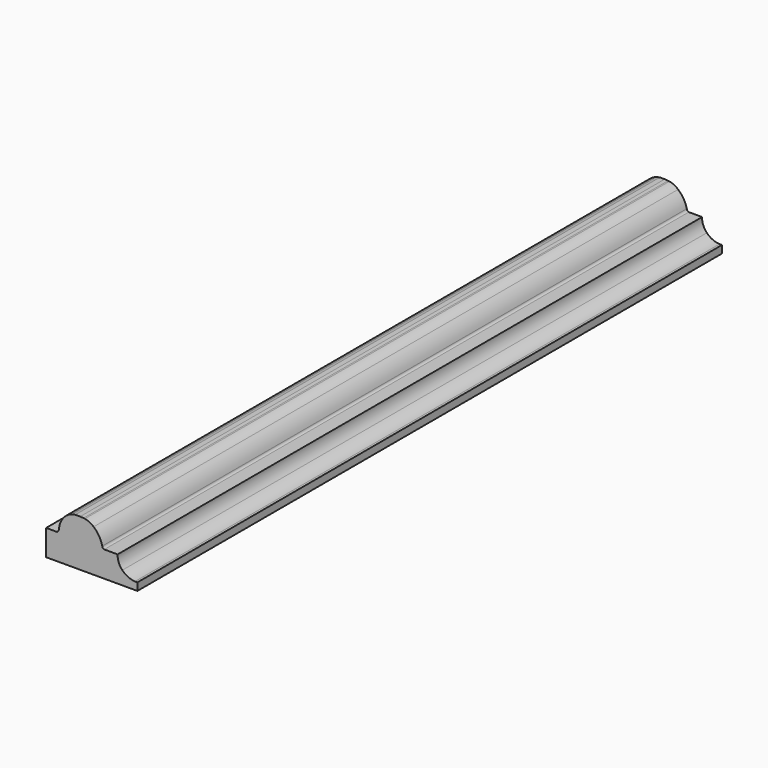
from build123d import *

# Parameters (mm, degrees)
F1_DEPTH = 152.4


# Not quite as in the source:
# - ends of sketch curves that miss each other by under 0.0002 mm in the source are joined


with BuildPart() as f1:
    # F0 (on Front) → F1 (new body)
    with BuildSketch(Plane.XZ):
        with BuildLine():
            Line((-9.525, 0.4953), (-9.525, -4.888738))
            Line((-9.525, -4.888738), (9.525, -4.8895))
            Line((9.525, -4.8895), (9.525, -3.3139888))
            Line((9.525, -3.3139888), (9.007348, -3.3139888))
            ThreePointArc((9.007348, -3.3139888), (7.5806290696, -2.9530541155), (6.3808590282, -2.1007851053))
            ThreePointArc((6.3808590282, -2.1007851053), (5.615744399, -0.9130091212), (5.3955415237, 0.4826001377))
            Line((5.3955415237, 0.4826001377), (2.6015442, 0.4826))
            ThreePointArc((2.6015442, 0.4826), (2.3116101055, 0.6590793559), (2.195162482, 0.9779044504))
            ThreePointArc((2.195162482, 0.9779044504), (1.5242441759, 2.5923195678), (0.3926111465, 3.92493888))
            ThreePointArc((0.3926111465, 3.92493888), (-0.4543047996, 4.4987348188), (-1.4312133596, 4.8023046334))
            Line((-1.4312133596, 4.8023046334), (-1.6949178252, 4.8349308979))
            Line((-1.6949178252, 4.8349308979), (-2.410714, 4.8895))
            Line((-2.410714, 4.8895), (-3.426714, 4.8895))
            Line((-3.426714, 4.8895), (-4.163314, 4.7117))
            Line((-4.163314, 4.7117), (-4.798314, 4.4577))
            Line((-4.798314, 4.4577), (-5.331714, 4.1021))
            ThreePointArc((-5.331714, 4.1021), (-6.256392611, 3.0214411434), (-6.7541092682, 1.6890991273))
            Line((-6.7541092682, 1.6890991273), (-6.881114, 0.9779))
            ThreePointArc((-6.881114, 0.9779), (-7.0732646412, 0.615608671), (-7.4653139443, 0.4953005843))
            Line((-7.4653139443, 0.4953005843), (-9.525, 0.4953))
        make_face()
    extrude(amount=F1_DEPTH)


solid = f1.part
